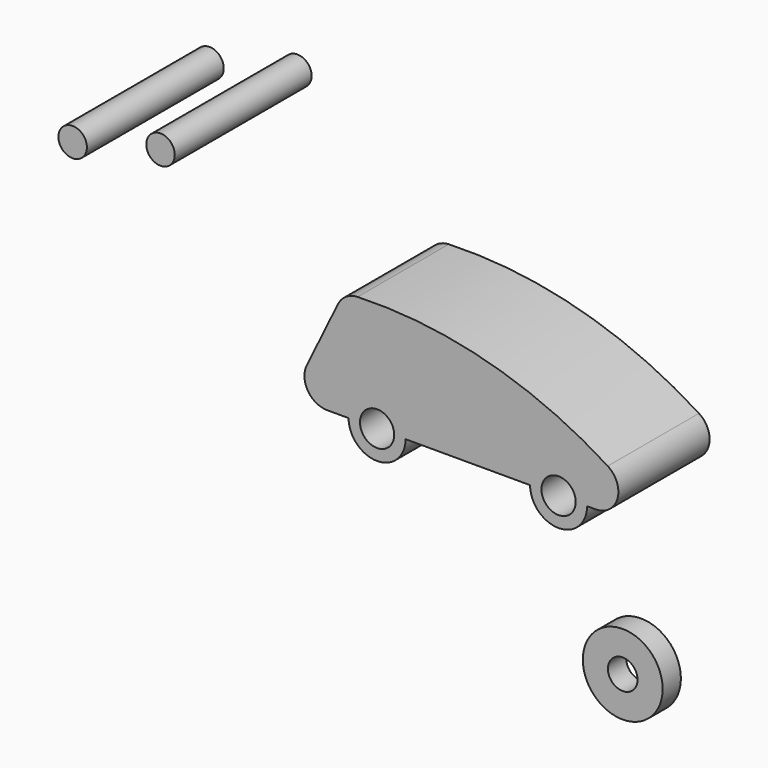
from build123d import *

# Parameters (mm, degrees)
F1_DEPTH    = 25.4
F2_T        = 2.54
F2_T3_DEPTH = 30.48
F3_R        = 12.5715428013
F4_DEPTH    = 25.4
F5_R        = 3.175
F6_DEPTH    = 38.1
F8_R        = 8.89
F8_R_2      = 3.302
F9_DEPTH    = 5.08
F10_R       = 5.9052801824
F11_DEPTH   = 29.464


# Not quite as in the source:
# - a shell that OpenCascade refuses in one call is made with other operations: the cavity is built on its own and cut out


with BuildPart() as f1:
    # F0 (on Front) → F1 (new body)
    with BuildSketch(Plane.XZ):
        with BuildLine():
            ThreePointArc((40.6837563911, 12.9512595013), (45.5633080309, 16.6183278701), (43.3981157839, 22.3252847791))
            ThreePointArc((43.3981157839, 22.3252847791), (16.6771448475, 34.0559195708), (-12.3172349893, 37.3640940343))
            ThreePointArc((-12.3172349893, 37.3640940343), (-14.9032820969, 36.5451200142), (-16.6991979645, 34.5121310115))
            Line((-16.6991979645, 34.5121310115), (-23.6436870624, 20.2559263329))
            ThreePointArc((-23.6436870624, 20.2559263329), (-23.3841308643, 15.3382043129), (-19.0767124086, 12.9512595013))
            Line((-19.0767124086, 12.9512595013), (-14.3209207639, 12.9512595013))
            ThreePointArc((-14.3209207639, 12.9512595013), (-7.9709207639, 19.3012595013), (-1.6209207639, 12.9512595013))
            Line((-1.6209207639, 12.9512595013), (26.098913902, 12.9512595013))
            ThreePointArc((26.098913902, 12.9512595013), (32.448913902, 19.3012595013), (38.798913902, 12.9512595013))
            Line((38.798913902, 12.9512595013), (40.6837563911, 12.9512595013))
        make_face()
        with BuildLine():
            ThreePointArc((26.098913902, 12.9512595013), (32.448913902, 6.6012595013), (38.798913902, 12.9512595013))
            Line((38.798913902, 12.9512595013), (36.258913902, 12.9512595013))
            ThreePointArc((36.258913902, 12.9512595013), (32.448913902, 9.1412595013), (28.638913902, 12.9512595013))
            Line((28.638913902, 12.9512595013), (26.098913902, 12.9512595013))
        make_face()
        with BuildLine():
            Line((36.258913902, 12.9512595013), (38.798913902, 12.9512595013))
            ThreePointArc((38.798913902, 12.9512595013), (32.448913902, 19.3012595013), (26.098913902, 12.9512595013))
            Line((26.098913902, 12.9512595013), (28.638913902, 12.9512595013))
            ThreePointArc((28.638913902, 12.9512595013), (32.448913902, 16.7612595013), (36.258913902, 12.9512595013))
        make_face()
        with BuildLine():
            ThreePointArc((-14.3209207639, 12.9512595013), (-7.9709207639, 6.6012595013), (-1.6209207639, 12.9512595013))
            Line((-1.6209207639, 12.9512595013), (-4.1609207639, 12.9512595013))
            ThreePointArc((-4.1609207639, 12.9512595013), (-7.9709207639, 9.1412595013), (-11.7809207639, 12.9512595013))
            Line((-11.7809207639, 12.9512595013), (-14.3209207639, 12.9512595013))
        make_face()
        with BuildLine():
            Line((-4.1609207639, 12.9512595013), (-1.6209207639, 12.9512595013))
            ThreePointArc((-1.6209207639, 12.9512595013), (-7.9709207639, 19.3012595013), (-14.3209207639, 12.9512595013))
            Line((-14.3209207639, 12.9512595013), (-11.7809207639, 12.9512595013))
            ThreePointArc((-11.7809207639, 12.9512595013), (-7.9709207639, 16.7612595013), (-4.1609207639, 12.9512595013))
        make_face()
    extrude(amount=F1_DEPTH)

    # F2: shell of thickness 2.54, made by hand


with BuildPart() as f2_core1:
    # F2_t2: copy of F1
    add(f1.part)

    # the walls: a layer under each face that stays
    f2_faces = [f2_core1.faces().sort_by_distance(p)[0] for p in [
        (45.5633080309, -12.7, 16.6183278701),
        (16.6771448475, -12.7, 34.0559195708),
        (-14.9032820969, -12.7, 36.5451200142),
        (-20.1714425135, -12.7, 27.3840286722),
        (-23.3841308643, -12.7, 15.3382043129),
        (-16.6988165863, -12.7, 12.9512595013),
        (-7.9709207639, -12.7, 6.6012595013),
        (12.2389965691, -12.7, 12.9512595013),
        (32.448913902, -12.7, 6.6012595013),
        (39.7413351466, -12.7, 12.9512595013),
        (28.638913902, -12.7, 12.9512595013),
        (-11.7809207639, -12.7, 12.9512595013),
        (10.8035219912, 0, 22.0150577288),
        (10.8035219912, -25.4, 22.0150577288),
    ]]
    thicken(f2_faces, amount=-F2_T, mode=Mode.SUBTRACT)

    # F2_s4 → F2_t3 (cut)
    with BuildSketch(Plane.XZ.offset(-2.54)):
        Polygon((-14.3463207639, 12.9258595013), (-14.3209207639, 15.4912595013), (-11.7809207639, 15.4912595013), (-11.7809207639, 12.9512595013), align=None)
        Polygon((-1.5955207639, 12.9258595013), (-4.1609207639, 12.9512595013), (-4.1609207639, 15.4912595013), (-1.6209207639, 15.4912595013), align=None)
        Polygon((26.073513902, 12.9258595013), (26.098913902, 15.4912595013), (28.638913902, 15.4912595013), (28.638913902, 12.9512595013), align=None)
        Polygon((38.824313902, 12.9258595013), (36.258913902, 12.9512595013), (36.258913902, 15.4912595013), (38.798913902, 15.4912595013), align=None)
    extrude(amount=F2_T3_DEPTH, mode=Mode.SUBTRACT)


with BuildPart() as f1_1:
    add(f1.part)

    # what is left inside the walls is the cavity
    f2_cavity = [f2_core1.part.solids().sort_by_distance(p)[0] for p in [
        (16.008612, -16.086667, 31.579159),
    ]]
    add(f2_cavity, mode=Mode.SUBTRACT)

    # F10 (on Right) → F11 (cut)
    with BuildSketch(Plane.YZ):
        with Locations((-12.3756462708, 27.3415483534)):
            Circle(F10_R)
    extrude(amount=-F11_DEPTH, mode=Mode.SUBTRACT)


with BuildPart() as f4:
    # F3 (on Front) → F4 (new body)
    with BuildSketch(Plane.XZ):
        with Locations((-40.8684164286, -40.0050021708)):
            Circle(F3_R)
    extrude(amount=F4_DEPTH)


with BuildPart() as f6:
    # F5 (on Front) → F6 (new body)
    with BuildSketch(Plane.XZ):
        with Locations((-65.6197145581, 55.5465146899)):
            Circle(F5_R)
    extrude(amount=F6_DEPTH)


with BuildPart() as f6b:
    # F5 (on Front) → F6, piece 2 (new body)
    with BuildSketch(Plane.XZ):
        with Locations((-46.0489206016, 60.4392103851)):
            Circle(F5_R)
    extrude(amount=F6_DEPTH)


with BuildPart() as f9:
    # F8 (on Front) → F9 (new body)
    with BuildSketch(Plane.XZ):
        with Locations((30.4775213926, -30.9622374706)):
            Circle(F8_R)
        with Locations((30.4775213926, -30.9622374706)):
            Circle(F8_R_2, mode=Mode.SUBTRACT)
    extrude(amount=F9_DEPTH)


solid = Compound([f1_1.part, f6.part, f6b.part, f9.part])
